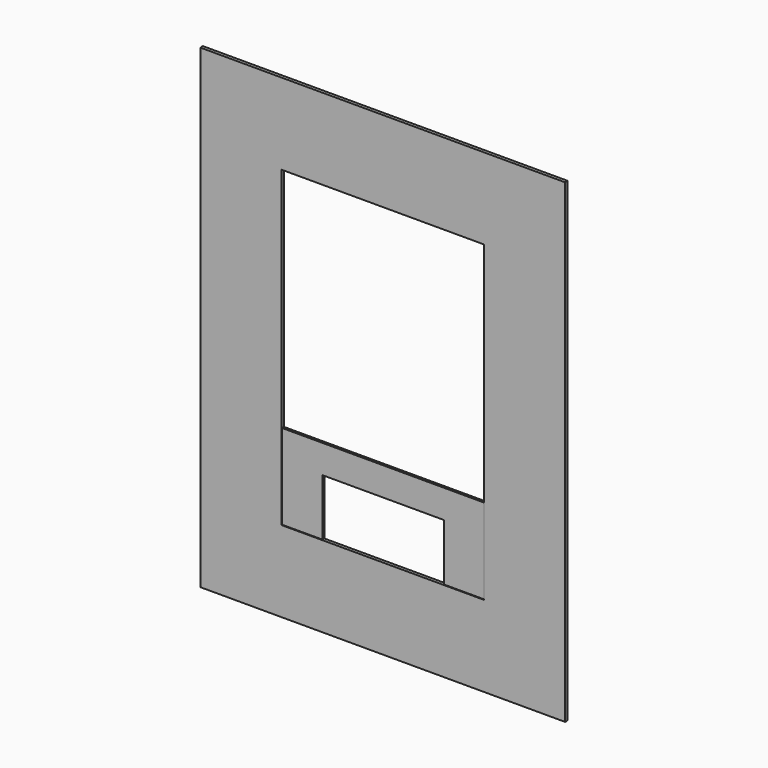
from build123d import *

# Parameters (mm, degrees)
F0_W     = 450
F0_H     = 586
F0_W_2   = 250
F0_H_2   = 386
F1_DEPTH = 4
F2_W     = 330
F2_H     = 466
F2_W_2   = 150
F2_H_2   = 70
F2_W_3   = 250
F2_H_3   = 281
F3_DEPTH = 3
F4_W     = 330
F4_H     = 466
F4_W_2   = 324
F4_H_2   = 460
F5_DEPTH = 31


with BuildPart() as f1:
    # F0 (on Front) → F1 (new body)
    with BuildSketch(Plane.XZ):
        with Locations((5.2358553946, 16.5430586814)):
            Rectangle(F0_W, F0_H)
        with Locations((5.2358553946, 16.5430586814)):
            Rectangle(F0_W_2, F0_H_2, mode=Mode.SUBTRACT)
    extrude(amount=F1_DEPTH)


with BuildPart() as f3:
    # F2 (on Front) → F3 (new body)
    with BuildSketch(Plane.XZ):
        with Locations((5.2358553946, 16.5430586814)):
            Rectangle(F2_W, F2_H)
        with Locations((5.2358553946, -141.4569413186)):
            Rectangle(F2_W_2, F2_H_2, mode=Mode.SUBTRACT)
        with Locations((5.2358553946, 69.0430586814)):
            Rectangle(F2_W_3, F2_H_3, mode=Mode.SUBTRACT)
    extrude(amount=F3_DEPTH)

    # F4 (on face) → F5 (join)
    with BuildSketch(Plane(origin=(0, 0, 0), x_dir=(-1, 0, 0), z_dir=(0, 1, 0))):
        with Locations((-5.2358553946, 16.5430586814)):
            Rectangle(F4_W, F4_H)
        with Locations((-5.2358553946, 16.5430586814)):
            Rectangle(F4_W_2, F4_H_2, mode=Mode.SUBTRACT)
    extrude(amount=F5_DEPTH)


solid = Compound([f1.part, f3.part])
